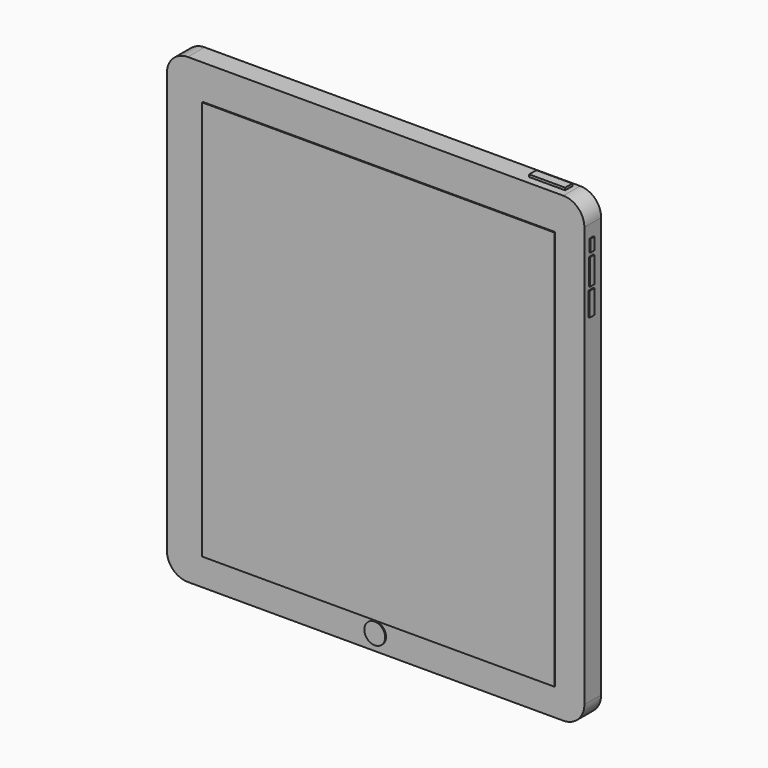
from build123d import *

# Parameters (mm, degrees)
F0_R      = 2.737762288
F0_R_2    = 1.0985637782
F1_DEPTH  = 5.08
F2_W      = 85.2321013808
F2_H      = 96.7953205109
F3_DEPTH  = 0.254
F6_DEPTH  = 93.3540835977
F5_R      = 1.9645563542
F5_R_2    = 1.7038978903
F5_R_3    = 1.5780003366
F5_R_4    = 1.5237356412
F7_W      = 8.7204426527
F7_H      = 2.1868101903
F8_DEPTH  = 0.5746809766
F9_R      = 2.5250145547
F10_DEPTH = 0.254
F11_W     = 1.3652069028
F11_H     = 6.2867105007
F11_W_2   = 1.403221162
F11_H_2   = 5.7247150689
F11_W_3   = 1.1607955676
F11_H_3   = 2.9349811375
F12_DEPTH = 0.254


# Not quite as in the source:
# - a feature names something its author has since deleted; it is built from what else it names


with BuildPart() as f1:
    # F0 (on Front) → F1 (new body)
    with BuildSketch(Plane.XZ):
        with BuildLine():
            Line((45.462447716, 55.951051414), (-45.462447716, 55.951051414))
            ThreePointArc((-45.462447716, 55.951051414), (-49.0545501644, 54.4631538624), (-50.542447716, 50.871051414))
            Line((-50.542447716, 50.871051414), (-50.542447716, -50.871051414))
            ThreePointArc((-50.542447716, -50.871051414), (-49.0545501644, -54.4631538624), (-45.462447716, -55.951051414))
            Line((-45.462447716, -55.951051414), (45.462447716, -55.951051414))
            ThreePointArc((45.462447716, -55.951051414), (49.0545501644, -54.4631538624), (50.542447716, -50.871051414))
            Line((50.542447716, -50.871051414), (50.542447716, 50.871051414))
            ThreePointArc((50.542447716, 50.871051414), (49.0545501644, 54.4631538624), (45.462447716, 55.951051414))
        make_face()
        with Locations((0, -50.8815050125)):
            Circle(F0_R, mode=Mode.SUBTRACT)
        with Locations((0, 50.8815050125)):
            Circle(F0_R_2, mode=Mode.SUBTRACT)
        with Locations((0, -50.8815050125)):
            Circle(F0_R)
        with Locations((0, 50.8815050125)):
            Circle(F0_R_2)
    extrude(amount=F1_DEPTH)

    # F2 (on face) → F3 (join)
    with BuildSketch(Plane.XZ.offset(5.08)):
        with Locations((0.8392669261, -0.8392669261)):
            Rectangle(F2_W, F2_H)
    extrude(amount=F3_DEPTH)

    # F7 (on face) → F8 (join)
    with BuildSketch(Plane.XY.offset(55.951051414)):
        with Locations((39.9978160858, -2.066604764)):
            Rectangle(F7_W, F7_H)
    extrude(amount=F8_DEPTH)

    # F9 (on face) → F10 (join)
    with BuildSketch(Plane.XZ.offset(5.08)):
        with Locations((0, -52.0344786346)):
            Circle(F9_R)
    extrude(amount=F10_DEPTH)

    # F11 (on face) → F12 (join)
    with BuildSketch(Plane.YZ.offset(50.542447716)):
        with Locations((-3.0571169918, 40.8467166126)):
            Rectangle(F11_W, F11_H)
        with Locations((-3.0761241214, 34.0065797791)):
            Rectangle(F11_W_2, F11_H_2)
        with Locations((-2.9549113242, 46.373186633)):
            Rectangle(F11_W_3, F11_H_3)
    extrude(amount=F12_DEPTH)


with BuildPart() as f6:
    # F4 (on face) → F6 (new body)
    with BuildSketch(Plane(origin=(0, 0, -55.951051414), x_dir=(1, 0, 0), z_dir=(0, 0, -1))):
        Polygon((6.1532426625, 3.1897546723), (-10.7177691534, 3.632507287), (-10.7177691534, 1.3415296562), (6.1532426625, 1.3415296562), align=None)
    extrude(amount=-F6_DEPTH)


with BuildPart() as f6b:
    # F5 (on face) → F6, piece 2 (new body)
    with BuildSketch(Plane(origin=(0, 0, -55.951051414), x_dir=(1, 0, 0), z_dir=(0, 0, -1))):
        with Locations((-40.9486070275, 2.4606343359)):
            Circle(F5_R)
    extrude(amount=-F6_DEPTH)


with BuildPart() as f6c:
    # F5 (on face) → F6, piece 3 (new body)
    with BuildSketch(Plane(origin=(0, 0, -55.951051414), x_dir=(1, 0, 0), z_dir=(0, 0, -1))):
        with Locations((-35.9550975263, 2.5903359056)):
            Circle(F5_R_2)
    extrude(amount=-F6_DEPTH)


with BuildPart() as f6d:
    # F5 (on face) → F6, piece 4 (new body)
    with BuildSketch(Plane(origin=(0, 0, -55.951051414), x_dir=(1, 0, 0), z_dir=(0, 0, -1))):
        with Locations((-31.1561413109, 2.5903359056)):
            Circle(F5_R_3)
    extrude(amount=-F6_DEPTH)


with BuildPart() as f6e:
    # F5 (on face) → F6, piece 5 (new body)
    with BuildSketch(Plane(origin=(0, 0, -55.951051414), x_dir=(1, 0, 0), z_dir=(0, 0, -1))):
        with Locations((-26.6165900975, 2.525486052)):
            Circle(F5_R_4)
    extrude(amount=-F6_DEPTH)


solid = Compound([f1.part, f6.part, f6b.part, f6c.part, f6d.part, f6e.part])
